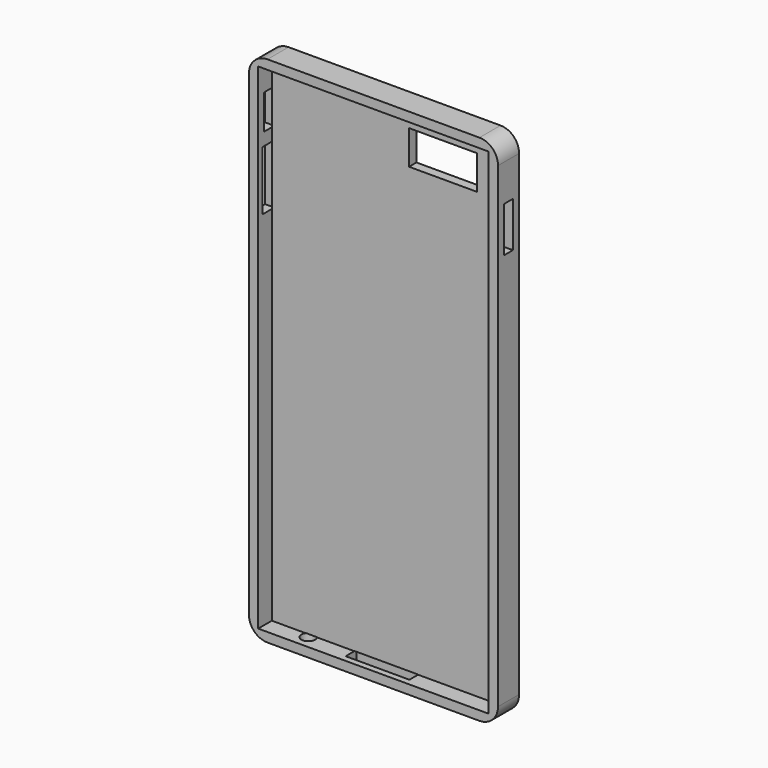
from build123d import *

# Parameters (mm, degrees)
F0_W      = 67.1
F0_H      = 138.3
F1_DEPTH  = 3.55
F2_T      = -2.5
F3_R      = 5
F4_W      = 18.3261586353
F4_H      = 9.162325412
F5_DEPTH  = 12.5
F6_W      = 17.1764912084
F6_H      = 3.6870999029
F7_DEPTH  = 2.55
F8_W      = 3.479784471
F8_H      = 9.3234963715
F9_DEPTH  = 2.55
F10_W     = 3.967121942
F10_H     = 15.9676056355
F11_DEPTH = 2.55
F12_R     = 1.8775227945
F13_DEPTH = 2.55
F17_W     = 2.9842249351
F17_H     = 12.1664553881
F18_DEPTH = 2.5


# Not quite as in the source:
# - the program builds the solid bodies; features that only make, move or delete a surface that nothing else refers to are left out


with BuildPart() as f1:
    # F0 (on Front) → F1 (new body, symmetric)
    with BuildSketch(Plane.XZ):
        Rectangle(F0_W, F0_H)
    extrude(amount=F1_DEPTH, both=True)

    # F2
    f2_openings = [f1.faces().sort_by_distance(p)[0] for p in [
        (0, -3.55, 0),
    ]]
    offset(amount=F2_T, openings=f2_openings)

    # F3
    f3_edges = [f1.edges().sort_by_distance(p)[0] for p in [
        (-33.55, 0, 69.15),
        (33.55, 0, 69.15),
        (-33.55, 0, -69.15),
        (33.55, 0, -69.15),
    ]]
    fillet(f3_edges, radius=F3_R)

    # F4 (on Front) → F5 (cut, symmetric)
    with BuildSketch(Plane.XZ):
        with Locations((15.0705915876, 57.5918015093)):
            Rectangle(F4_W, F4_H)
    extrude(amount=F5_DEPTH, both=True, mode=Mode.SUBTRACT)

    # F6 (on face) → F7 (cut, symmetric)
    with BuildSketch(Plane(origin=(0, 0, -69.15), x_dir=(1, 0, 0), z_dir=(0, 0, -1))):
        with Locations((-0.2433923073, 0.0339728431)):
            Rectangle(F6_W, F6_H)
    extrude(amount=F7_DEPTH, both=True, mode=Mode.SUBTRACT)

    # F8 (on face) → F9 (cut, symmetric)
    with BuildSketch(Plane(origin=(-33.55, 0, 0), x_dir=(0, -1, 0), z_dir=(-1, 0, 0))):
        with Locations((-0.1312090899, 55.0323408097)):
            Rectangle(F8_W, F8_H)
    extrude(amount=F9_DEPTH, both=True, mode=Mode.SUBTRACT)

    # F10 (on face) → F11 (cut, symmetric)
    with BuildSketch(Plane(origin=(-33.55, 0, 0), x_dir=(0, -1, 0), z_dir=(-1, 0, 0))):
        with Locations((0.1124596456, 38.9681095257)):
            Rectangle(F10_W, F10_H)
    extrude(amount=F11_DEPTH, both=True, mode=Mode.SUBTRACT)

    # F12 (on face) → F13 (cut, symmetric)
    with BuildSketch(Plane(origin=(0, 0, -69.15), x_dir=(1, 0, 0), z_dir=(0, 0, -1))):
        with Locations((-20.385697484, 0)):
            Circle(F12_R)
    extrude(amount=F13_DEPTH, both=True, mode=Mode.SUBTRACT)

    # F17 (on face) → F18 (cut, symmetric)
    with BuildSketch(Plane.YZ.offset(33.55)):
        with Locations((-0.036496378, 48.1377318501)):
            Rectangle(F17_W, F17_H)
    extrude(amount=F18_DEPTH, both=True, mode=Mode.SUBTRACT)


solid = f1.part
